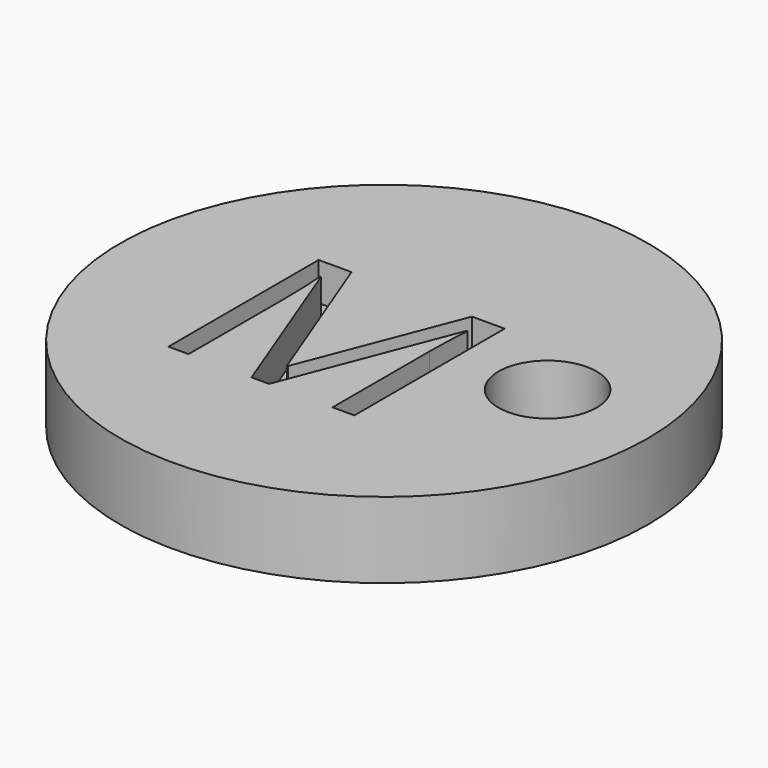
from build123d import *

# Parameters (mm, degrees)
F0_R         = 34.7443251371
F1_DEPTH     = 10
F2_R         = 6.463042093
F3_DEPTH     = 10
F4_TEXT_SIZE = 34.6318585798
F5_DEPTH     = 5


# Not quite as in the source:
# - Text() gives the source's letters only with a copy of the font that has no kerning and outlines rounded to 1/6400 em; it was checked with that copy


with BuildPart() as f1:
    # F0 (on Top) → F1 (new body)
    with BuildSketch(Plane.XY):
        with Locations((-97.1056371927, 34.3686975539)):
            Circle(F0_R)
    extrude(amount=F1_DEPTH)

    # F2 (on face) → F3 (cut)
    with BuildSketch(Plane.XY.offset(10)):
        with Locations((-77.2037729621, 36.3948941231)):
            Circle(F2_R)
    extrude(amount=-F3_DEPTH, mode=Mode.SUBTRACT)

    # F4 (on face) → F5 (cut)
    with BuildSketch(Plane.XY.offset(10)):
        with Locations((-117.0029863715, 19.4986704737)):
            Text('M', F4_TEXT_SIZE, font='Open Sans', text_align=(TextAlign.LEFT, TextAlign.BOTTOM))
    extrude(amount=-F5_DEPTH, mode=Mode.SUBTRACT)


solid = f1.part
